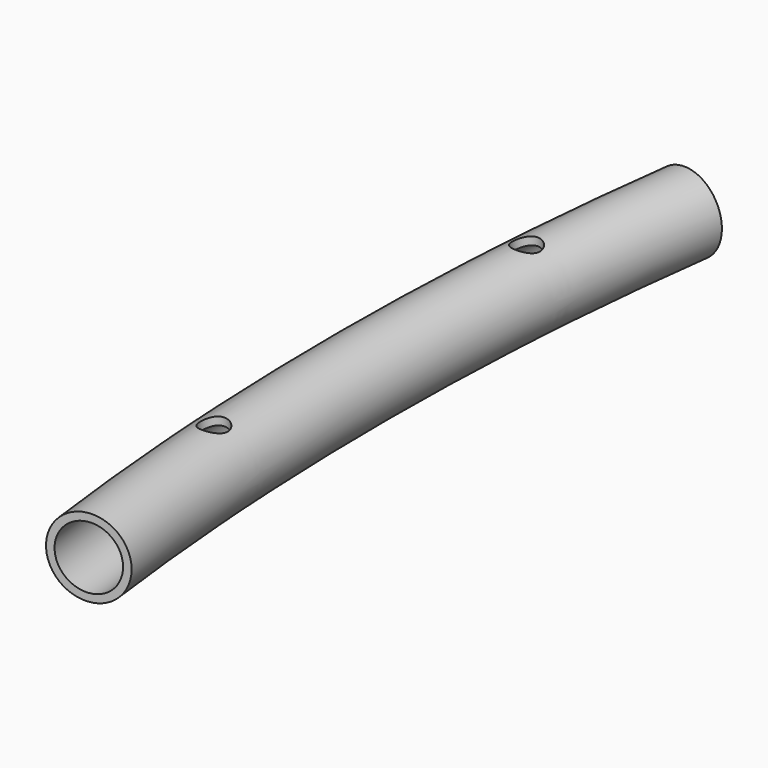
from build123d import *
from build123d import SkipClean  # not in build123d's __all__

# Parameters (mm, degrees)
F0_R          = 15
F0_R_2        = 12
F1_ANGLE_BACK = 7.5
F1_ANGLE      = 15
F2_R          = 5.25
F3_DEPTH      = 15.001
F3_DEPTH_BACK = 15.001


with BuildPart() as f1:
    # F0 (on Front) → F1 (revolve)
    with BuildSketch(Plane.XZ, mode=Mode.PRIVATE) as f1_sk:
        with Locations((-1100, 0)):
            Circle(F0_R)
        with Locations((-1100, 0)):
            Circle(F0_R_2, mode=Mode.SUBTRACT)
    revolve(f1_sk.sketch.rotate(Axis((0, 0, 190.0846064091), (0, 0, -1)), -F1_ANGLE_BACK), axis=Axis((0, 0, 190.0846064091), (0, 0, -1)), revolution_arc=F1_ANGLE)

    # F2 (on Top) → F3 (cut, two sides)
    with BuildSketch(Plane.XY) as f3_sk:
        with Locations((-1097.4402033824, -75)):
            Circle(F2_R)
        with Locations((-1097.4402033824, 75)):
            Circle(F2_R)
    with SkipClean():  # cleaning this boolean's faces spoils the solid; the shape is the same uncleaned
        extrude(amount=-F3_DEPTH, mode=Mode.SUBTRACT)
        extrude(f3_sk.sketch, amount=F3_DEPTH_BACK, mode=Mode.SUBTRACT)


solid = f1.part
